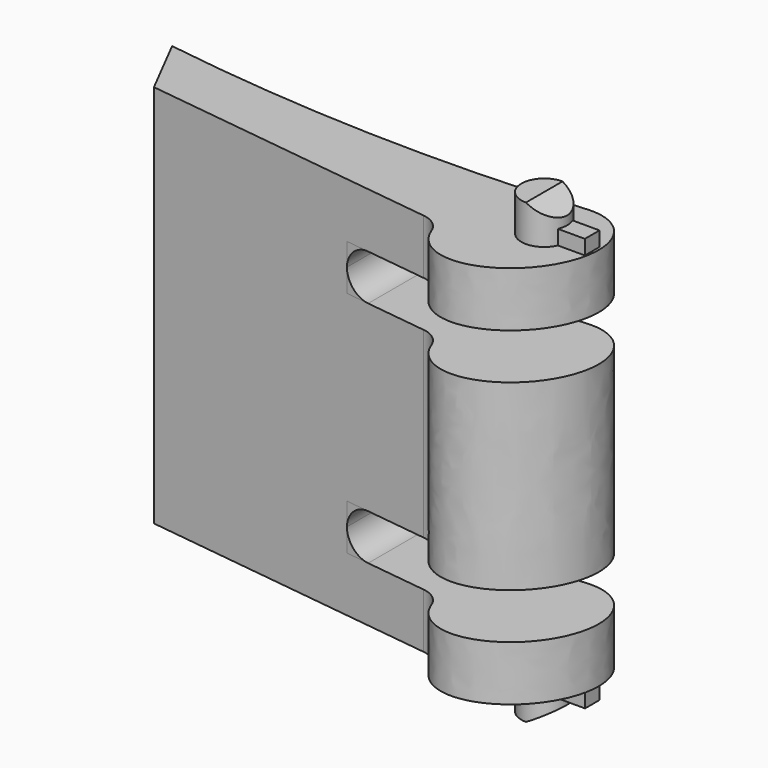
from build123d import *

# Parameters (mm, degrees)
F1_DEPTH     = 21
F3_W         = 15.0982862345
F3_H         = 25.1671721393
F4_DEPTH     = 2.5
F6_W         = 27.927816356
F6_H         = 22.3754025899
F7_DEPTH     = 2.5
F8_T4_DEPTH  = 10.3582394023
F8_S5_R      = 100
F8_T6_DEPTH  = 7
F8_T11_DEPTH = 10.3582394023
F8_S12_R     = 100
F8_T13_DEPTH = 7
F8_T18_DEPTH = 10.3582394023
F8_S19_R     = 100
F8_T20_DEPTH = 7
F8_T25_DEPTH = 10.3582394023
F8_S26_R     = 100
F8_T27_DEPTH = 7
F9_R         = 1.4
F10_R        = 1.25
F11_DEPTH    = 2
F13_R        = 1.25
F14_DEPTH    = 2
F17_W        = 1.492921263
F17_H        = 4.4254288077
F18_DEPTH    = 25
F21_W        = 1.9132951934
F21_H        = 3.2676104456
F22_DEPTH    = 25
F23_W        = 2.6214234531
F23_H        = 1
F24_DEPTH    = 0.8
F25_W        = 2.6302933693
F25_H        = 1
F26_DEPTH    = 0.8


# Not quite as in the source:
# - a fillet or chamfer that OpenCascade refuses, or shapes differently, is made with other operations: its cross-section is extruded or revolved along the edge and cut away or added


with BuildPart() as f1:
    # F0 (on Top) → F1 (new body)
    with BuildSketch(Plane.XY):
        with BuildLine():
            Line((25.7519837469, 30.1143433899), (43.1284420192, 27.9130078852))
            add(Edge.make_bspline(
                [(43.1284420192, 27.9130078852), (43.748237159, 21.1619048692), (48.845124386, 27.2907595332), (53.9420116129, 33.4196141972), (47.2293113268, 32.8441807488)],
                knots=[2.4902540559, 2.4902540559, 2.4902540559, 4.7016901225, 4.7016901225, 6.9131261892, 6.9131261892, 6.9131261892], degree=2, weights=[1, 0.4484927805, 1, 0.4484927805, 1]))
            ThreePointArc((47.2293113268, 32.8441807488), (35.5868846063, 32.5268772196), (23.9865279377, 33.5653889592))
            Line((23.9865279377, 33.5653889592), (25.7519837469, 30.1143433899))
        make_face()
    extrude(amount=F1_DEPTH)

    # F3 (on offset) → F4 (cut)
    with BuildSketch(Plane.XY.offset(18)):
        with Locations((45.0356710549, 29.340852052)):
            Rectangle(F3_W, F3_H)
    extrude(amount=-F4_DEPTH, mode=Mode.SUBTRACT)

    # F6 (on offset) → F7 (cut)
    with BuildSketch(Plane(origin=(0, 0, 3), x_dir=(1, 0, 0), z_dir=(0, 0, -1))):
        with Locations((51.4504361157, -29.4867381454)):
            Rectangle(F6_W, F6_H)
    extrude(amount=-F7_DEPTH, mode=Mode.SUBTRACT)

    # F8: fillet of radius 1.3 on 4 edges, made by hand


with BuildPart() as f8_tool2:
    # F8_s3 → F8_t4 (new body)
    with BuildSketch(Plane.XZ.offset(-25.3777534097)):
        with BuildLine():
            ThreePointArc((38.7865279377, 5.5), (37.8672891221, 5.1192388155), (37.4865279377, 4.2))
            Line((37.4865279377, 4.2), (37.4865279377, 5.5))
            Line((37.4865279377, 5.5), (38.7865279377, 5.5))
        make_face()
    extrude(amount=-F8_T4_DEPTH)

    # F8_s5 → F8_t6 (cut, symmetric)
    with BuildSketch(Plane.XY.offset(4.8)):
        with Locations((38.6883258238, 132.4787709604)):
            Circle(F8_S5_R)
    extrude(amount=F8_T6_DEPTH, both=True, mode=Mode.SUBTRACT)

    split(bisect_by=Plane(origin=(4.1615402697, 32.8495273406, 0), x_dir=(0, 0, 1), z_dir=(0.1256804232, 0.9920707793, 0)), keep=Keep.TOP)


with BuildPart() as f1_1:
    add(f1.part)

    # F8_t1: union F8_tool2
    add(f8_tool2.part)


with BuildPart() as f8_tool9:
    # F8_s10 → F8_t11 (new body)
    with BuildSketch(Plane.XZ.offset(-35.735992812)):
        with BuildLine():
            ThreePointArc((38.7865279377, 18), (37.8672891221, 17.6192388155), (37.4865279377, 16.7))
            Line((37.4865279377, 16.7), (37.4865279377, 18))
            Line((37.4865279377, 18), (38.7865279377, 18))
        make_face()
    extrude(amount=F8_T11_DEPTH)

    # F8_s12 → F8_t13 (cut, symmetric)
    with BuildSketch(Plane.XY.offset(17.4)):
        with Locations((38.6883258238, 132.4787709604)):
            Circle(F8_S12_R)
    extrude(amount=F8_T13_DEPTH, both=True, mode=Mode.SUBTRACT)

    split(bisect_by=Plane(origin=(4.1615402697, 32.8495273406, 0), x_dir=(0, 0, 1), z_dir=(0.1256804232, 0.9920707793, 0)), keep=Keep.TOP)


with BuildPart() as f1_2:
    add(f1_1.part)

    # F8_t8: union F8_tool9
    add(f8_tool9.part)


with BuildPart() as f8_tool16:
    # F8_s17 → F8_t18 (new body)
    with BuildSketch(Plane.XZ.offset(-25.3777534097)):
        with BuildLine():
            ThreePointArc((37.4865279377, 4.3), (37.8672891221, 3.3807611845), (38.7865279377, 3))
            Line((38.7865279377, 3), (37.4865279377, 3))
            Line((37.4865279377, 3), (37.4865279377, 4.3))
        make_face()
    extrude(amount=-F8_T18_DEPTH)

    # F8_s19 → F8_t20 (cut, symmetric)
    with BuildSketch(Plane.XY.offset(3.7)):
        with Locations((38.6883258238, 132.4787709604)):
            Circle(F8_S19_R)
    extrude(amount=F8_T20_DEPTH, both=True, mode=Mode.SUBTRACT)

    split(bisect_by=Plane(origin=(4.1615402697, 32.8495273406, 0), x_dir=(0, 0, 1), z_dir=(0.1256804232, 0.9920707793, 0)), keep=Keep.TOP)


with BuildPart() as f1_3:
    add(f1_2.part)

    # F8_t15: union F8_tool16
    add(f8_tool16.part)


with BuildPart() as f8_tool23:
    # F8_s24 → F8_t25 (new body)
    with BuildSketch(Plane.XZ.offset(-35.735992812)):
        with BuildLine():
            ThreePointArc((37.4865279377, 16.8), (37.8672891221, 15.8807611845), (38.7865279377, 15.5))
            Line((38.7865279377, 15.5), (37.4865279377, 15.5))
            Line((37.4865279377, 15.5), (37.4865279377, 16.8))
        make_face()
    extrude(amount=F8_T25_DEPTH)

    # F8_s26 → F8_t27 (cut, symmetric)
    with BuildSketch(Plane.XY.offset(16.2)):
        with Locations((38.6883258238, 132.4787709604)):
            Circle(F8_S26_R)
    extrude(amount=F8_T27_DEPTH, both=True, mode=Mode.SUBTRACT)

    split(bisect_by=Plane(origin=(4.1615402697, 32.8495273406, 0), x_dir=(0, 0, 1), z_dir=(0.1256804232, 0.9920707793, 0)), keep=Keep.TOP)


with BuildPart() as f1_4:
    add(f1_3.part)

    # F8_t22: union F8_tool23
    add(f8_tool23.part)

    # F9
    f9_edges = [f1_4.edges().sort_by_distance(p)[0] for p in [
        (43.128442, 27.913008, 19.5),
        (43.128442, 27.913008, 10.5),
        (43.128442, 27.913008, 1.5),
    ]]
    fillet(f9_edges, radius=F9_R)

    # F10 (on face) → F11 (join)
    with BuildSketch(Plane.XY.offset(21)):
        with Locations((47.2179576755, 29.9575272948)):
            Circle(F10_R)
    extrude(amount=F11_DEPTH)

    # F13 (on face) → F14 (join)
    with BuildSketch(Plane(origin=(0, 0, 0), x_dir=(1, 0, 0), z_dir=(0, 0, -1))):
        with Locations((47.2179576755, -29.9575272948)):
            Circle(F13_R)
    extrude(amount=F14_DEPTH)

    # F17 (on line) → F18 (cut)
    with BuildSketch(Plane(origin=(12.6705148226, 0, -21.9459754309), x_dir=(0.8660254038, 0, 0.5), z_dir=(-0.5, 0, 0.8660254038))):
        with Locations((40.6311545521, 30.2472934127)):
            Rectangle(F17_W, F17_H)
    extrude(amount=-F18_DEPTH, mode=Mode.SUBTRACT)

    # F21 (on line) → F22 (cut)
    with BuildSketch(Plane(origin=(21.7637815624, 0, 37.6959754309), x_dir=(0.8660254038, 0, -0.5), z_dir=(-0.5, 0, -0.8660254038))):
        with Locations((30.3485984584, -30.0394026563)):
            Rectangle(F21_W, F21_H)
    extrude(amount=-F22_DEPTH, mode=Mode.SUBTRACT)

    # F23 (on face) → F24 (join)
    with BuildSketch(Plane.XY.offset(21)):
        with Locations((48.528669402, 29.9575272948)):
            Rectangle(F23_W, F23_H)
    extrude(amount=F24_DEPTH)

    # F25 (on face) → F26 (join)
    with BuildSketch(Plane(origin=(0, 0, 0), x_dir=(1, 0, 0), z_dir=(0, 0, -1))):
        with Locations((48.5331043601, -29.9575272948)):
            Rectangle(F25_W, F25_H)
    extrude(amount=F26_DEPTH)


solid = f1_4.part
